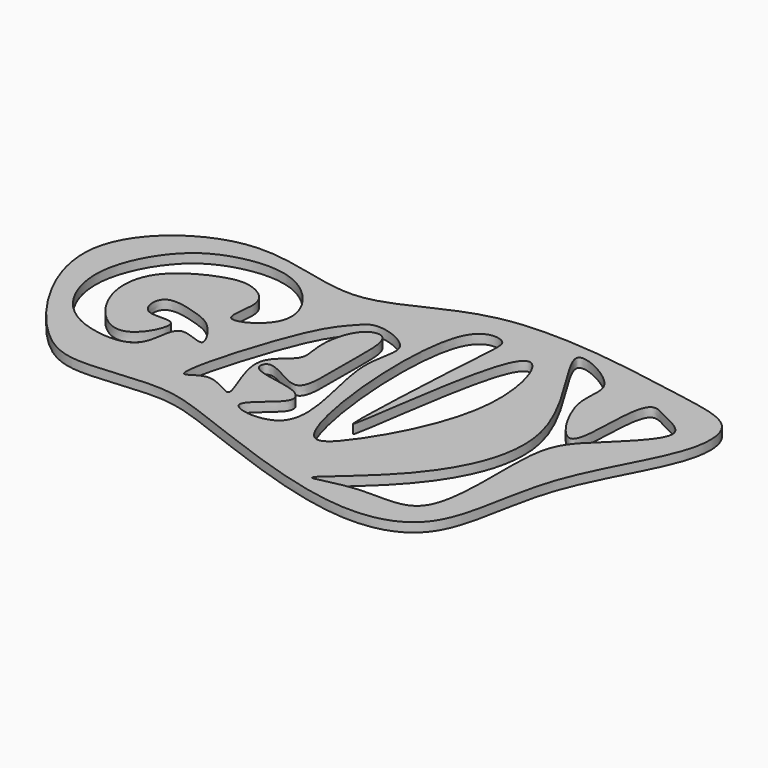
from build123d import *

# Parameters (mm, degrees)
F1_DEPTH = 5
F3_SCALE = 0.23


# Not quite as in the source:
# - a feature names something its author has since deleted; it is built from what else it names


with BuildPart() as f1:
    # F0 (on Top) → F1 (new body)
    with BuildSketch(Plane.XY):
        with BuildLine():
            add(Edge.make_bspline(
                [(299.1526722908, 323.0784237385), (274.741297579, 317.7973106885), (241.6552621715, 288.3027220251), (174.6561440066, 324.4303302875), (100.8407748129, 268.4649814376), (156.7674642815, 186.3116869244), (185.7324239145, 178.5277009697), (226.1707484356, 185.3868960132), (256.0578422928, 176.6418628219), (348.0516956151, 138.1310389921), (403.8224652859, 152.4437889707), (404.1484862835, 221.437686785), (441.7834657542, 274.608521823), (440.4545733731, 309.8452976444), (400.1148772466, 316.2758146237), (330.3168429715, 329.8204245647), (299.1526722908, 323.0784237385)],
                knots=[0, 0, 0, 0, 0.0765098554, 0.1538063765, 0.232258661, 0.3185876279, 0.3708037843, 0.4288031062, 0.4838122847, 0.5788917757, 0.6439585446, 0.7189607313, 0.796776055, 0.8454986106, 0.9023256076, 1, 1, 1, 1], degree=3))
        make_face()
        with BuildLine():
            add(Edge.make_bspline(
                [(226.7263020449, 199.5824126484), (223.4576288788, 202.786391877), (242.1999725363, 266.5677697188), (254.9145889572, 278.8865041127), (262.2909315988, 288.3151160053), (290.8198837548, 277.7046283826), (274.3932370472, 253.1572964006), (304.9409766216, 182.6462111975), (249.2001381077, 189.2102738309), (282.2021647662, 207.2813126016), (273.0104797985, 219.5491142599), (244.7923070222, 219.8121758246), (249.5684914386, 234.1886770838), (276.8869616896, 210.4946765653), (273.6219951966, 248.512588351), (276.7354158182, 282.053506119), (259.2033811273, 279.3122075457), (253.762364876, 255.811330661), (260.1649557791, 240.1490025527), (236.0654816291, 231.1378453304), (261.5056115576, 187.1467772907), (236.7501491374, 209.3350521643), (228.0747030749, 198.2606993193), (226.7263020449, 199.5824126484)],
                knots=[0, 0, 0, 0, 0.0828937124, 0.1308044326, 0.162120507, 0.209668973, 0.2608236325, 0.3408590433, 0.3905134761, 0.4381462453, 0.470498726, 0.5218879901, 0.5458835427, 0.5938746477, 0.6467827945, 0.7047251559, 0.7363843276, 0.7852002992, 0.8240810053, 0.8679177748, 0.9244345861, 0.9658044835, 1, 1, 1, 1], degree=3))
        make_face(mode=Mode.SUBTRACT)
        with BuildLine():
            add(Edge.make_bspline(
                [(209.8892042679, 269.8180302978), (208.7391356913, 275.6904528202), (198.2996826517, 282.1228271055), (184.4603080574, 280.7879675176), (154.881065232, 266.2225276434), (153.5011906417, 232.3077326247), (183.0296869747, 202.8430171081), (200.5101768899, 238.9914929912), (175.9333386204, 229.9797622421), (173.4325463009, 252.7590006492), (196.2162419723, 246.5162755468), (207.3140331244, 242.1999747822), (220.5981134819, 220.7979000543), (195.2467628131, 236.7300207175), (199.6007343954, 205.4106041471), (170.5913017144, 204.9089331269), (147.341051391, 217.3252499023), (135.0289416593, 250.412145169), (152.2943006175, 286.015422634), (177.499382771, 299.9227596674), (214.2694685831, 301.4527181362), (239.9833012028, 263.595362143), (203.5262003375, 244.0591017529), (211.1221596549, 263.5223752981), (209.8892042679, 269.8180302978)],
                knots=[0, 0, 0, 0, 0.0380651676, 0.0740988442, 0.1265193827, 0.1803922784, 0.2333369623, 0.2774756756, 0.3142296108, 0.3483184172, 0.3887194127, 0.4269446592, 0.4629599231, 0.4988968041, 0.5412781193, 0.5870720719, 0.6364206556, 0.6910847872, 0.7495727059, 0.8005680131, 0.8572782298, 0.9141073466, 0.9591914305, 1, 1, 1, 1], degree=3))
        make_face(mode=Mode.SUBTRACT)
        with BuildLine():
            add(Edge.make_bspline(
                [(298.3174920082, 302.3189604282), (302.6997885354, 310.2313695533), (316.914777746, 309.6989205916), (315.0880893818, 294.5653440912), (307.2984114695, 150.554089505), (321.9774488212, 289.0746952033), (338.4053423789, 307.6769167334), (354.0074026958, 255.0484992427), (325.3854707834, 199.7493760856), (297.29510477, 171.5239700843), (286.6295899339, 281.2159925089), (298.3174920082, 302.3189604282)],
                knots=[0, 0, 0, 0, 0.0671618297, 0.1342935011, 0.2885453965, 0.4394658231, 0.5059876178, 0.6135217323, 0.7521623528, 0.8208745383, 1, 1, 1, 1], degree=3))
        make_face(mode=Mode.SUBTRACT)
        with BuildLine():
            add(Edge.make_bspline(
                [(372.602917254, 304.0657788515), (367.4411923009, 311.0944849221), (326.8209510066, 331.53281104), (401.3140745104, 248.3245923877), (360.4250959964, 183.2250523588), (318.0265408159, 152.8555238781), (352.3695619063, 166.3020741455), (394.9323531346, 155.3824192087), (384.2421996806, 238.9066187979), (400.1111024667, 257.3689215259), (433.3189122381, 287.0655246284), (412.0651962212, 296.1954629907), (399.2583506311, 304.2206475385), (396.4259826336, 281.424061096), (397.0614821118, 240.9163112112), (369.1074517704, 285.2091693505), (377.1958170977, 297.8116403016), (372.602917254, 304.0657788515)],
                knots=[0, 0, 0, 0, 0.0609975824, 0.1595570064, 0.263227794, 0.3302440429, 0.3846953289, 0.4524289392, 0.5485219976, 0.6116810214, 0.6805869671, 0.7276284801, 0.7665743202, 0.8193722618, 0.8785679043, 0.9457243869, 1, 1, 1, 1], degree=3))
        make_face(mode=Mode.SUBTRACT)
    extrude(amount=F1_DEPTH)


with BuildPart() as f1_1:
    # F3: moved
    add(f1.part.scale(F3_SCALE).moved(Location((35.1951662451, 30.7942508906, 0))))


solid = f1_1.part
